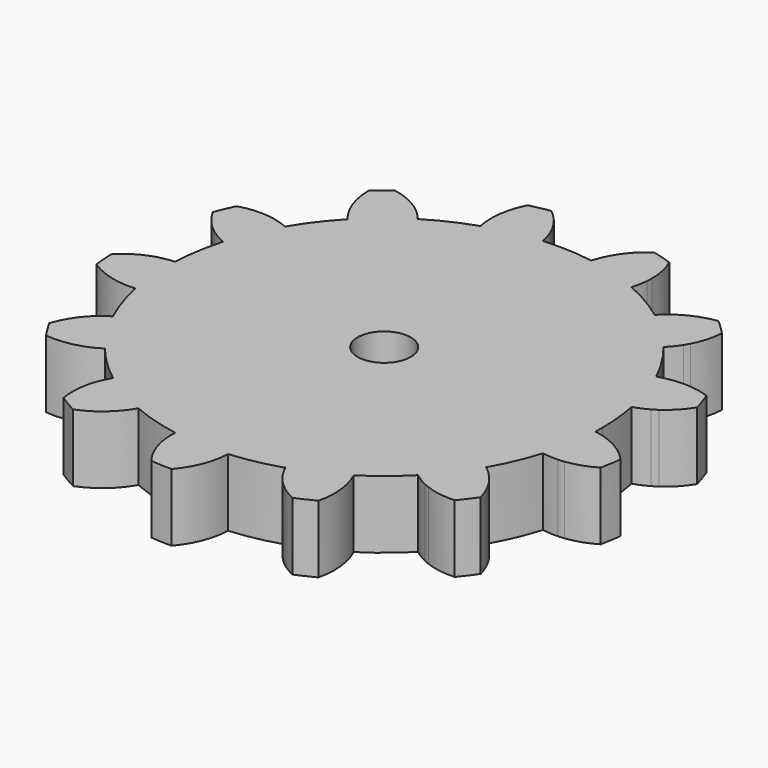
from build123d import *

# Parameters (mm, degrees)
F1_DEPTH = 6.35
F2_COUNT = 13
F3_R     = 2.5
F4_DEPTH = 6.351


with BuildPart() as f1:
    # F0 (on Top) → F1 (new body)
    with BuildSketch(Plane.XY):
        with BuildLine():
            ThreePointArc((7.9296197565, 23.5951858335), (6.9911317973, 23.8900761864), (6.0417249702, 24.1476546146))
            ThreePointArc((6.0417249702, 24.1476546146), (4.3226425573, 22.4330749308), (3.2648662162, 20.2476374354))
            ThreePointArc((3.2648662162, 20.2476374354), (5.7837443287, 19.6767495961), (8.2108987358, 18.7938105523))
            ThreePointArc((8.2108987358, 18.7938105523), (8.3954934616, 19.5156536929), (8.4994507341, 20.2534379554))
            ThreePointArc((8.4994507341, 20.2534379554), (8.5176465567, 20.5391701676), (8.5237154667, 20.8254168329))
            ThreePointArc((8.5237154667, 20.8254168329), (8.373521449, 22.2418004346), (7.9296197565, 23.5951858335))
        make_face()
        with BuildLine():
            ThreePointArc((4.0264902572, 14.4598933509), (-1.7431476836, 15.057566034), (-4.9211585336, 19.9100068261))
            ThreePointArc((-4.9211585336, 19.9100068261), (-12.6431262329, -16.1486077476), (20.5091729021, 0))
            ThreePointArc((20.5091729021, 0), (19.2415803806, 7.0984334598), (15.5954927821, 13.3194135761))
            ThreePointArc((15.5954927821, 13.3194135761), (9.5256046991, 10.9946956396), (4.0264902572, 14.4598933509))
        make_face()
        with BuildLine():
            ThreePointArc((3.2648662162, 20.2476374354), (-0.8451772993, 20.4917507417), (-4.9211585336, 19.9100068261))
            ThreePointArc((-4.9211585336, 19.9100068261), (-1.7431476836, 15.057566034), (4.0264902572, 14.4598933509))
            ThreePointArc((4.0264902572, 14.4598933509), (3.0384725246, 17.2738616412), (3.2648662162, 20.2476374354))
        make_face()
        with BuildLine():
            ThreePointArc((4.0264902572, 14.4598933509), (9.5256046991, 10.9946956396), (15.5954927821, 13.3194135761))
            ThreePointArc((15.5954927821, 13.3194135761), (12.2138579016, 16.4756744411), (8.2108987358, 18.7938105523))
            ThreePointArc((8.2108987358, 18.7938105523), (6.6287005247, 16.1344397874), (4.0264902572, 14.4598933509))
        make_face()
        with BuildLine():
            ThreePointArc((8.2108987358, 18.7938105523), (5.7837443287, 19.6767495961), (3.2648662162, 20.2476374354))
            ThreePointArc((3.2648662162, 20.2476374354), (3.0384725246, 17.2738616412), (4.0264902572, 14.4598933509))
            ThreePointArc((4.0264902572, 14.4598933509), (6.6287005247, 16.1344397874), (8.2108987358, 18.7938105523))
        make_face()
    extrude(amount=F1_DEPTH)

    # F2: F1 ×13 about axis
    f2_axis = Axis((0, 0, 6.35), (0, 0, 1))


with BuildPart() as f1_1:
    add(f1.part)
    for i in range(1, F2_COUNT):
        add(f1.part.rotate(f2_axis, i * 360 / F2_COUNT))

    # F3 (on face) → F4 (cut, through all)
    with BuildSketch(Plane.XY.offset(6.35)):
        Circle(F3_R)
    extrude(amount=-F4_DEPTH, mode=Mode.SUBTRACT)


solid = f1_1.part
